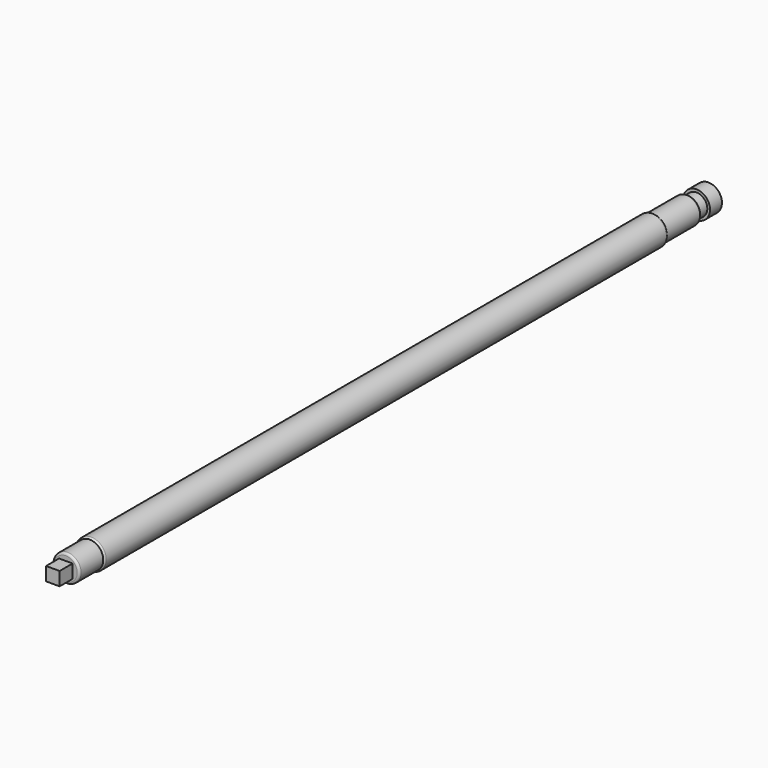
from build123d import *

# Parameters (mm, degrees)
F0_R      = 34.925
F1_DEPTH  = 825.5
F2_R      = 31.75
F3_DEPTH  = 69.85
F4_R      = 31.75
F5_DEPTH  = 101.6
F6_W      = 31.75
F6_H      = 31.75
F7_DEPTH  = 38.1
F8_R      = 25.4
F9_DEPTH  = 25.4
F10_R     = 31.75
F10_R_2   = 25.4
F11_DEPTH = 34.925
F14_DEPTH = 6.35


# Not quite as in the source:
# - a fillet or chamfer that OpenCascade refuses, or shapes differently, is made with other operations: its cross-section is extruded or revolved along the edge and cut away or added


with BuildPart() as f1:
    # F0 (on Front) → F1 (new body, symmetric)
    with BuildSketch(Plane.XZ):
        Circle(F0_R)
    extrude(amount=F1_DEPTH, both=True)

    # F2 (on face) → F3 (join)
    with BuildSketch(Plane.XZ.offset(825.5)):
        Circle(F2_R)
    extrude(amount=F3_DEPTH)

    # F4 (on face) → F5 (join)
    with BuildSketch(Plane(origin=(0, 825.5, 0), x_dir=(-1, 0, 0), z_dir=(0, 1, 0))):
        Circle(F4_R)
    extrude(amount=F5_DEPTH)

    # F6 (on face) → F7 (join)
    with BuildSketch(Plane.XZ.offset(895.35)):
        Rectangle(F6_W, F6_H)
    extrude(amount=F7_DEPTH)

    # F8 (on face) → F9 (join)
    with BuildSketch(Plane(origin=(0, 927.1, 0), x_dir=(-1, 0, 0), z_dir=(0, 1, 0))):
        Circle(F8_R)
    extrude(amount=F9_DEPTH)

    # F10 (on face) → F11 (join)
    with BuildSketch(Plane(origin=(0, 952.5, 0), x_dir=(-1, 0, 0), z_dir=(0, 1, 0))):
        Circle(F10_R)
        Circle(F10_R_2, mode=Mode.SUBTRACT)
        Circle(F10_R_2)
    extrude(amount=F11_DEPTH)

    # F12: fillet of radius 5.08 on 4 edges, made by hand

    # F12_s1 → F12_t2 (revolve, cut)
    with BuildSketch(Plane.XY):
        with BuildLine():
            ThreePointArc((31.75, 825.5), (34.0571134838, 823.6305202921), (34.925, 820.7907139607))
            Line((34.925, 820.7907139607), (34.925, 825.5))
            Line((34.925, 825.5), (31.75, 825.5))
        make_face()
    revolve(axis=Axis((0, 825.5, 0), (0, -1, 0)), mode=Mode.SUBTRACT)

    # F12_s3 → F12_t4 (revolve, cut)
    with BuildSketch(Plane.XY):
        with BuildLine():
            ThreePointArc((34.925, -820.7907139607), (34.0571134838, -823.6305202921), (31.75, -825.5))
            Line((31.75, -825.5), (34.925, -825.5))
            Line((34.925, -825.5), (34.925, -820.7907139607))
        make_face()
    revolve(axis=Axis((0, -825.5, 0), (0, -1, 0)), mode=Mode.SUBTRACT)

    # F12_s5 → F12_t6 (revolve, cut)
    with BuildSketch(Plane.XY):
        with BuildLine():
            ThreePointArc((31.75, -890.27), (30.2621024484, -893.8621024484), (26.67, -895.35))
            Line((26.67, -895.35), (31.75, -895.35))
            Line((31.75, -895.35), (31.75, -890.27))
        make_face()
    revolve(axis=Axis((0, -895.35, 0), (0, -1, 0)), mode=Mode.SUBTRACT)

    # F12_s7 → F12_t8 (revolve, cut)
    with BuildSketch(Plane.XY):
        with BuildLine():
            ThreePointArc((-26.67, 927.1), (-30.2621024484, 925.6121024484), (-31.75, 922.02))
            Line((-31.75, 922.02), (-31.75, 927.1))
            Line((-31.75, 927.1), (-26.67, 927.1))
        make_face()
    revolve(axis=Axis((0, 927.1, 0), (0, 1, 0)), mode=Mode.SUBTRACT)

    # F13 (on face) → F14 (cut)
    with BuildSketch(Plane(origin=(0, 987.425, 0), x_dir=(-1, 0, 0), z_dir=(0, 1, 0))):
        Polygon((2.749630657, 4.7625), (-2.749630657, 4.7625), (-5.499261314, 0), (-2.749630657, -4.7625), (2.749630657, -4.7625), (5.499261314, 0), align=None)
    extrude(amount=-F14_DEPTH, mode=Mode.SUBTRACT)


solid = f1.part
